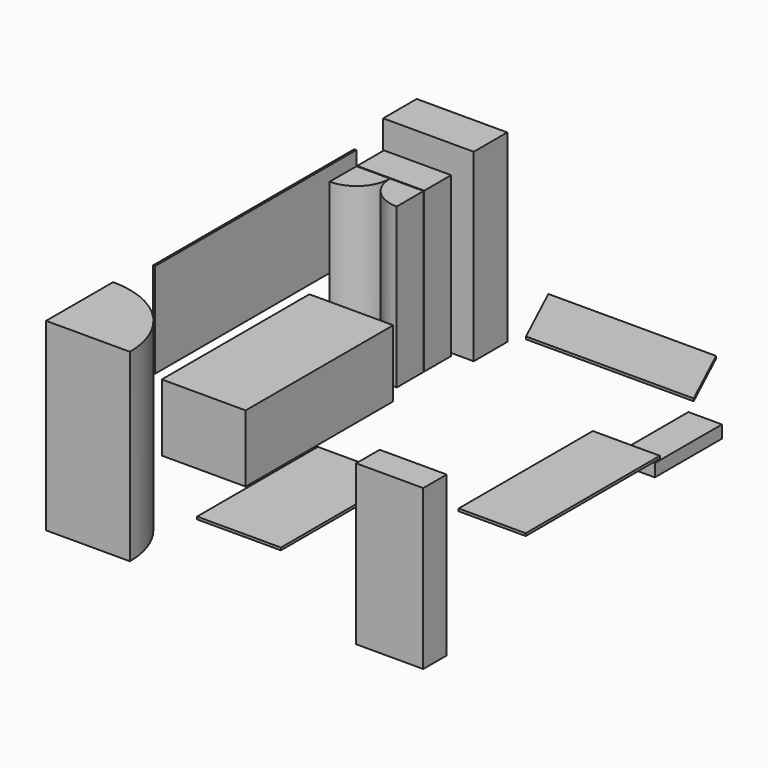
from build123d import *

# Parameters (mm, degrees)
F5_DEPTH  = 2200
F1_W      = 1080
F1_H      = 500
F6_DEPTH  = 2200
F7_START  = 700
F4_W      = 800
F4_H      = 2000
F7_DEPTH  = 30
F8_START  = 450
F4_W_2    = 400
F4_H_2    = 1000
F8_DEPTH  = 150
F9_START  = 700
F2_W      = 1000
F2_H      = 1200
F2_H_2    = 600
F9_DEPTH  = 30
F11_START = 700
F11_DEPTH = 30
F12_W     = 3000
F12_H     = 1130
F13_DEPTH = 25
F10_W     = 1000
F10_H     = 2200
F14_DEPTH = 800
F15_W     = 800
F15_H     = 400
F16_DEPTH = 1900
F15_H_2   = 350
F18_DEPTH = 1900


# Not quite as in the source:
# - a feature names something its author has since deleted; it is built from what else it names


with BuildPart() as f5:
    # F3 (on Top) → F5 (new body)
    with BuildSketch(Plane.XY):
        with BuildLine():
            Line((100, 0), (1100, 0))
            ThreePointArc((1100, 0), (807.1067811865, 707.1067811865), (100, 1000))
            Line((100, 1000), (100, 0))
        make_face()
    extrude(amount=F5_DEPTH)


with BuildPart() as f6:
    # F1 (on Top) → F6 (new body)
    with BuildSketch(Plane.XY):
        with Locations((540, 5400)):
            Rectangle(F1_W, F1_H)
    extrude(amount=F6_DEPTH)


with BuildPart() as f7:
    # F4 (on Top) → F7 (new body)
    with BuildSketch(Plane.XY.offset(F7_START)):
        with Locations((4100, 2650)):
            Rectangle(F4_W, F4_H)
    extrude(amount=F7_DEPTH)


with BuildPart() as f8:
    # F4 (on Top) → F8 (new body)
    with BuildSketch(Plane.XY.offset(F8_START)):
        with Locations((4200, 4200)):
            Rectangle(F4_W_2, F4_H_2)
    extrude(amount=F8_DEPTH)


with BuildPart() as f9:
    # F2 (on Top) → F9 (new body)
    with BuildSketch(Plane.XY.offset(F9_START)):
        with Locations((2400, 601)):
            Rectangle(F2_W, F2_H)
        with Locations((2400, 1501)):
            Rectangle(F2_W, F2_H_2)
    extrude(amount=F9_DEPTH)


with BuildPart() as f11:
    # F4 (on Top) → F11 (new body)
    with BuildSketch(Plane.XY.offset(F11_START)):
        Polygon((3650, 5550), (1650, 5550), (2023.046126524, 4750), (4023.046126524, 4750), align=None)
    extrude(amount=F11_DEPTH)


with BuildPart() as f13:
    # F12 (on Right) → F13 (new body)
    with BuildSketch(Plane.YZ):
        with Locations((3250, 1465)):
            Rectangle(F12_W, F12_H)
    extrude(amount=-F13_DEPTH)


with BuildPart() as f14:
    # F10 (on Top) → F14 (new body)
    with BuildSketch(Plane.XY):
        with Locations((500, 2950)):
            Rectangle(F10_W, F10_H)
    extrude(amount=F14_DEPTH)


with BuildPart() as f16:
    # F15 (on Top) → F16 (new body)
    with BuildSketch(Plane.XY):
        with Locations((450, 4900)):
            Rectangle(F15_W, F15_H)
    extrude(amount=F16_DEPTH)


with BuildPart() as f16b:
    # F15 (on Top) → F16, piece 2 (new body)
    with BuildSketch(Plane.XY):
        with Locations((4190, 185)):
            Rectangle(F15_W, F15_H_2)
    extrude(amount=F16_DEPTH)


with BuildPart() as f18:
    # F17 (on Top) → F18 (new body)
    with BuildSketch(Plane.XY):
        with BuildLine():
            Line((850, 4690), (450, 4690))
            ThreePointArc((450, 4690), (567.1572875254, 4407.1572875254), (850, 4290))
            Line((850, 4290), (850, 4690))
        make_face()
    extrude(amount=F18_DEPTH)

    # F17 (on Top) → F18, piece 2 (join)
    with BuildSketch(Plane.XY):
        with BuildLine():
            Line((450, 4690), (50, 4690))
            Line((50, 4690), (50, 4290))
            ThreePointArc((50, 4290), (332.8427124746, 4407.1572875254), (450, 4690))
        make_face()
    extrude(amount=F18_DEPTH)


solid = Compound([f5.part, f6.part, f7.part, f8.part, f9.part, f11.part, f13.part, f14.part, f16.part, f16b.part, f18.part])
